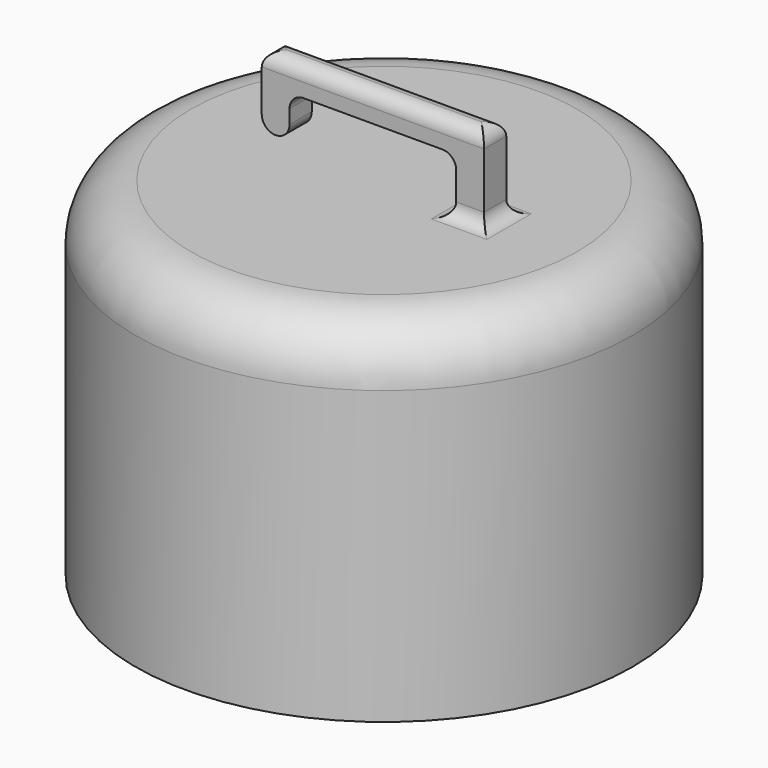
from build123d import *

# Parameters (mm, degrees)
F0_R     = 17.9
F0_R_2   = 16.5
F1_DEPTH = 25
F3_DEPTH = 2
F4_W     = 2
F4_H     = 3
F4_H_2   = 2
F5_DEPTH = 1
F6_R     = 0.99999
F7_R     = 4
F8_SIZE2 = 0.1099571106
F8_SIZE  = 18


# Not quite as in the source:
# - a fillet or chamfer is up to 0.001 mm smaller than in the source, because OpenCascade refuses the exact size


with BuildPart() as f1:
    # F0 (on Top) → F1 (new body)
    with BuildSketch(Plane.XY):
        Circle(F0_R)
        Circle(F0_R_2, mode=Mode.SUBTRACT)
    extrude(amount=-F1_DEPTH)

    # F0 (on Top) → F3 (join)
    with BuildSketch(Plane.XY):
        Circle(F0_R_2)
    extrude(amount=-F3_DEPTH)

    # F4 (on face) → F5 (join, symmetric)
    with BuildSketch(Plane.XZ):
        Polygon((6, 4), (6, 0), (8, 0), (8, 6), (6, 6), align=None)
        with Locations((-7, 2.5)):
            Rectangle(F4_W, F4_H)
        with Locations((-7, 5)):
            Rectangle(F4_W, F4_H_2)
        Polygon((-4, 4), (6, 4), (6, 6), (-6, 6), (-6, 4), align=None)
    extrude(amount=F5_DEPTH, both=True)

    # F6 (radius 1 in the source; OpenCascade refuses exactly that, so slightly less here)
    f6_edges = [f1.edges().sort_by_distance(p)[0] for p in [
        (8, 0, 0),
        (7, -1, 0),
        (7, 1, 0),
        (6, 0, 4),
        (-6, 0, 4),
        (8, 0, 6),
        (-8, 0, 6),
        (6, 0, 0),
        (-8, 0, 1),
        (-6, 0, 1),
        (0, -1, 6),
        (0, 1, 6),
    ]]
    fillet(f6_edges, radius=F6_R)

    # F7
    f7_edges = [f1.edges().sort_by_distance(p)[0] for p in [
        (-17.9, 0, 0),
        (-16.5, 0, -2),
    ]]
    fillet(f7_edges, radius=F7_R)

    # F8
    f8_edges = [f1.edges().sort_by_distance(p)[0] for p in [
        (-16.5, 0, -25),
    ]]
    f8_side = f1.faces().sort_by_distance((-16.5, 0, -15.5))[0]
    chamfer(f8_edges, length=F8_SIZE, length2=F8_SIZE2, reference=f8_side)


solid = f1.part
